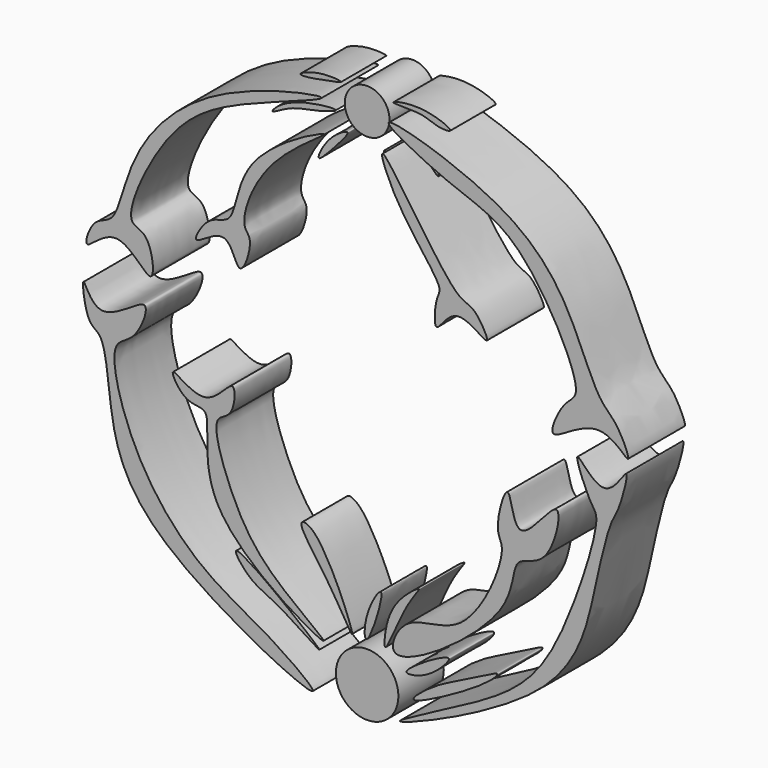
from build123d import *

# Parameters (mm, degrees)
F3_R      = 2.2031193739
F4_DEPTH  = 4
F5_R      = 1.5762828789
F6_DEPTH  = 4
F8_DEPTH  = 5
F13_DEPTH = 5
F14_DEPTH = 5
F15_DEPTH = 5
F19_DEPTH = 5
F20_DEPTH = 5
F21_DEPTH = 5
F22_DEPTH = 5
F29_DEPTH = 4
F30_DEPTH = 4
F31_DEPTH = 4
F32_DEPTH = 4
F33_DEPTH = 4
F34_DEPTH = 4
F39_DEPTH = 4
F40_DEPTH = 4
F41_DEPTH = 4
F42_DEPTH = 4
F45_DEPTH = 4
F46_DEPTH = 4


# Not quite as in the source:
# - the program builds the solid bodies; features that only make, move or delete a surface that nothing else refers to are left out


with BuildPart() as f4:
    # F3 (on Front) → F4 (new body)
    with BuildSketch(Plane.XZ):
        with Locations((0, 2.3418962955)):
            Circle(F3_R)
    extrude(amount=F4_DEPTH)


with BuildPart() as f6:
    # F5 (on Front) → F6 (new body)
    with BuildSketch(Plane.XZ):
        with Locations((0, 37.9213877022)):
            Circle(F5_R)
    extrude(amount=F6_DEPTH)


with BuildPart() as f8:
    # F7 (on Front) → F8 (new body)
    with BuildSketch(Plane.XZ):
        with BuildLine():
            add(Edge.make_bspline(
                [(2.8010457754, 5.6113414466), (3.7490480342, 5.0526232335), (11.660464427, 10.3387411352), (10.7959679961, 14.559460332), (13.7441495824, 14.2067494477), (15.0188095178, 20.4242651347), (11.155763458, 14.1209353977), (10.8886984205, 19.9195584963), (9.6547685549, 15.3268691163), (10.8927378391, 14.7424811012), (7.938159407, 7.593573555), (3.4600012996, 8.6814348962), (2.339180326, 5.8835482227), (2.8010457754, 5.6113414466)],
                knots=[0, 0, 0, 0, 0.1497805879, 0.2426028863, 0.3147246339, 0.4039610203, 0.4935151706, 0.5675421593, 0.6465099561, 0.7028059861, 0.826898522, 0.9270270952, 1, 1, 1, 1], degree=3))
        make_face()
    extrude(amount=F8_DEPTH)


with BuildPart() as f13:
    # F10 (on Front) → F13 (new body)
    with BuildSketch(Plane.XZ):
        with BuildLine():
            add(Edge.make_bspline(
                [(-3.0461507849, 1.3452416752), (-3.4818464728, 1.0746526722), (-15.9466824959, 7.0883957863), (-17.3440535719, 14.0645430033), (-17.6964457302, 18.7752133758), (-19.0105397095, 18.8901683902), (-19.4788265599, 22.8417380605), (-18.2227719071, 18.7192140814), (-13.9632338729, 22.9603577053), (-15.5052584544, 18.8233068375), (-17.6905007654, 18.6818873374), (-15.8132900001, 11.5879474918), (-10.9962366401, 6.1504658227), (-6.6372556078, 4.254425972), (-2.8057086264, 1.4945683859), (-3.0461507849, 1.3452416752)],
                knots=[0, 0, 0, 0, 0.1339251424, 0.241594644, 0.3161355758, 0.3560233968, 0.412737319, 0.4636841603, 0.5330688457, 0.5898577481, 0.638861131, 0.7327648109, 0.8364260377, 0.9260923364, 1, 1, 1, 1], degree=3))
        make_face()
    extrude(amount=F13_DEPTH)


with BuildPart() as f14:
    # F11 (on Front) → F14 (new body)
    with BuildSketch(Plane.XZ):
        with BuildLine():
            add(Edge.make_bspline(
                [(-2.2868220694, 4.7186701559), (-2.6059892866, 4.6507073984), (-12.0999546825, 9.7755638468), (-9.7225185843, 16.8469305379), (-12.0622915375, 16.1343630453), (-13.6245494081, 18.964401828), (-10.4806569975, 15.9435882622), (-8.3487910491, 19.617965915), (-8.5830237681, 16.343588236), (-10.4412698192, 16.3521021675), (-8.5839180053, 10.8751642204), (-6.1482469705, 7.5075225049), (-2.0830393164, 4.7620632021), (-2.2868220694, 4.7186701559)],
                knots=[0, 0, 0, 0, 0.1554468363, 0.2749627788, 0.3349269565, 0.3990039473, 0.4767777833, 0.5543183117, 0.6195590867, 0.6743415246, 0.7823936617, 0.9007498811, 1, 1, 1, 1], degree=3))
        make_face()
    extrude(amount=F14_DEPTH)


with BuildPart() as f15:
    # F12 (on Front) → F15 (new body)
    with BuildSketch(Plane.XZ):
        with BuildLine():
            add(Edge.make_bspline(
                [(3.1202319078, 1.4828173444), (3.4277099811, 1.3932976165), (15.1813481771, 6.1176914834), (16.6875533637, 13.5859063631), (17.8983054266, 18.7917910272), (18.5481634415, 19.4361719166), (19.5950481907, 23.4514253732), (17.598851761, 19.2728908312), (14.8574838152, 23.4901190525), (16.5072711493, 19.2369526839), (17.3805448102, 18.7408839057), (15.1014088235, 11.5459960258), (12.3522853152, 6.5322070241), (7.4192099097, 3.8040285678), (2.9342883779, 1.5369532833), (3.1202319078, 1.4828173444)],
                knots=[0, 0, 0, 0, 0.1271530156, 0.2380593294, 0.3201159226, 0.3626020469, 0.4205450423, 0.4754452226, 0.533326587, 0.5942311074, 0.6345672285, 0.7337673076, 0.8273503335, 0.9231057997, 1, 1, 1, 1], degree=3))
        make_face()
    extrude(amount=F15_DEPTH)


with BuildPart() as f19:
    # F18 (on Front) → F19 (new body)
    with BuildSketch(Plane.XZ):
        with BuildLine():
            add(Edge.make_bspline(
                [(2.322970191, 38.3718237281), (2.5270910425, 38.7261250095), (11.9414135575, 36.0254427021), (15.4403073522, 30.293092001), (17.0726428574, 25.8587327004), (18.4737587842, 25.0532840335), (19.7867006527, 21.928521176), (17.1824421043, 25.4080690427), (12.990501005, 21.4406454045), (14.6318823595, 25.2767119865), (16.4303038149, 25.7301784196), (11.7448821367, 34.6297607631), (7.2388170198, 35.5260575644), (2.1717541082, 38.1093515136), (2.322970191, 38.3718237281)],
                knots=[0, 0, 0, 0, 0.1221092671, 0.2379537302, 0.323282405, 0.3794516036, 0.4358004654, 0.4993232222, 0.5769736094, 0.6387431351, 0.688165312, 0.8080616155, 0.9095394473, 1, 1, 1, 1], degree=3))
        make_face()
    extrude(amount=F19_DEPTH)


with BuildPart() as f20:
    # F17 (on Front) → F20 (new body)
    with BuildSketch(Plane.XZ):
        with BuildLine():
            add(Edge.make_bspline(
                [(1.9492642023, 36.2945869565), (2.5109444115, 35.9835217607), (6.9870378528, 28.5395111667), (8.2735961106, 29.1699334606), (10.0407799206, 26.0465320892), (6.971187526, 29.0233585074), (5.4286092857, 25.7134326681), (5.5973243084, 28.6806268497), (6.3325602319, 29.3568256566), (2.8897882043, 33.0379384873), (1.6250355459, 36.4741486516), (1.9492642023, 36.2945869565)],
                knots=[0, 0, 0, 0, 0.2013367397, 0.2860860069, 0.3773616619, 0.480397428, 0.5740353547, 0.6631838563, 0.7269218084, 0.8837788131, 1, 1, 1, 1], degree=3))
        make_face()
    extrude(amount=F20_DEPTH)


with BuildPart() as f21:
    # F16 (on Front) → F21 (new body)
    with BuildSketch(Plane.XZ):
        with BuildLine():
            add(Edge.make_bspline(
                [(-2.4252030998, 38.3797101676), (-2.4789846343, 38.5840722079), (-10.8069291148, 36.8788326973), (-16.0797222373, 30.7867074955), (-16.7930252537, 25.7173030694), (-18.5509802615, 25.8142728569), (-19.4827202682, 22.8675548903), (-16.7471027116, 26.3270879047), (-13.9220735744, 21.7701284075), (-14.4697933803, 26.2085478406), (-16.7366984942, 25.9222789509), (-13.3311489117, 33.4451286462), (-8.560655082, 36.1864951779), (-2.3784401481, 38.2020177249), (-2.4252030998, 38.3797101676)],
                knots=[0, 0, 0, 0, 0.1142575183, 0.2418402879, 0.3288066955, 0.3788868359, 0.4314786293, 0.4961302535, 0.5681089731, 0.6329376534, 0.6802608121, 0.787273635, 0.9006532842, 1, 1, 1, 1], degree=3))
        make_face()
    extrude(amount=F21_DEPTH)


with BuildPart() as f22:
    # F9 (on Front) → F22 (new body)
    with BuildSketch(Plane.XZ):
        with BuildLine():
            add(Edge.make_bspline(
                [(-2.2471314296, 36.1804254353), (-2.4297902392, 36.2355529609), (-8.5531195322, 33.3510451306), (-8.3437817698, 28.2841304607), (-10.4221559056, 28.6321210069), (-11.986198059, 25.7036030989), (-8.902264517, 28.6096428837), (-8.2729905956, 24.6368009538), (-7.1236667489, 28.0723362786), (-8.3168221546, 28.5557775169), (-6.683407476, 33.4905561644), (-2.0860682132, 36.1318155894), (-2.2471314296, 36.1804254353)],
                knots=[0, 0, 0, 0, 0.1469308705, 0.2724688016, 0.3476298065, 0.4252506236, 0.5116434508, 0.5939968645, 0.6788859293, 0.7369512488, 0.8704406393, 1, 1, 1, 1], degree=3))
        make_face()
    extrude(amount=F22_DEPTH)


with BuildPart() as f29:
    # F25 (on Front) → F29 (new body)
    with BuildSketch(Plane.XZ):
        with BuildLine():
            add(Edge.make_bspline(
                [(-1.8493793905, 39.138160646), (-1.8212072767, 39.2195451719), (-3.3926815622, 39.3771778296), (-5.3397557879, 38.5319502967), (-3.4896675647, 38.7516512444), (-2.9207049201, 38.9460915409), (-1.8713033434, 39.0748260119), (-1.8493793905, 39.138160646)],
                knots=[0, 0, 0, 0, 0.229458845, 0.4515464705, 0.6414348687, 0.8214317548, 1, 1, 1, 1], degree=3))
        make_face()
    extrude(amount=F29_DEPTH)


with BuildPart() as f30:
    # F26 (on Front) → F30 (new body)
    with BuildSketch(Plane.XZ):
        with BuildLine():
            add(Edge.make_bspline(
                [(-2.2203600965, 37.2760854661), (-2.2482048938, 37.3740834609), (-4.3006399089, 37.1876575574), (-6.1438132913, 36.4548829278), (-6.9987236159, 35.4434833858), (-5.3279235742, 36.5584028629), (-3.5918143504, 36.7183597714), (-2.1977171419, 37.196395026), (-2.2203600965, 37.2760854661)],
                knots=[0, 0, 0, 0, 0.1813484263, 0.3912494782, 0.4973853163, 0.650377817, 0.8525302895, 1, 1, 1, 1], degree=3))
        make_face()
    extrude(amount=F30_DEPTH)


with BuildPart() as f31:
    # F27 (on Front) → F31 (new body)
    with BuildSketch(Plane.XZ):
        with BuildLine():
            add(Edge.make_bspline(
                [(-1.3842144981, 36.1581631005), (-1.4654348488, 36.2598773586), (-2.8320166984, 35.4910009057), (-3.8049234588, 33.3224757949), (-2.3854156249, 34.8318687171), (-1.2984933507, 36.0508123832), (-1.3842144981, 36.1581631005)],
                knots=[0, 0, 0, 0, 0.247607324, 0.5036170042, 0.7386716047, 1, 1, 1, 1], degree=3))
        make_face()
    extrude(amount=F31_DEPTH)


with BuildPart() as f32:
    # F24 (on Front) → F32 (new body)
    with BuildSketch(Plane.XZ):
        with BuildLine():
            add(Edge.make_bspline(
                [(1.2257457711, 35.8971096575), (1.3447218931, 35.9440675201), (2.3119158995, 34.5374387809), (2.3400667486, 32.9646713994), (1.9558439298, 34.006873836), (1.439716885, 34.8077793744), (1.1374107412, 35.8622453156), (1.2257457711, 35.8971096575)],
                knots=[0, 0, 0, 0, 0.2498050049, 0.4532304733, 0.5993389115, 0.8145297375, 1, 1, 1, 1], degree=3))
        make_face()
    extrude(amount=F32_DEPTH)


with BuildPart() as f33:
    # F28 (on Front) → F33 (new body)
    with BuildSketch(Plane.XZ):
        with BuildLine():
            add(Edge.make_bspline(
                [(1.854308648, 39.066825062), (1.7829226729, 39.1471854731), (3.7626423728, 39.6518215727), (6.5607006963, 38.5445827834), (4.8477423703, 38.5270656292), (3.9337949577, 39.1324017282), (1.9249394007, 38.9873148177), (1.854308648, 39.066825062)],
                knots=[0, 0, 0, 0, 0.2162198195, 0.4547725674, 0.5953127328, 0.7860676614, 1, 1, 1, 1], degree=3))
        make_face()
    extrude(amount=F33_DEPTH)


with BuildPart() as f34:
    # F23 (on Front) → F34 (new body)
    with BuildSketch(Plane.XZ):
        with BuildLine():
            add(Edge.make_bspline(
                [(2.4007428437, 37.5778712332), (2.4898800691, 37.6262023146), (4.923256046, 36.5808170939), (5.1721828368, 35.106890813), (4.2680461742, 36.4346272144), (2.3199123661, 37.5340441523), (2.4007428437, 37.5778712332)],
                knots=[0, 0, 0, 0, 0.3154577662, 0.4986855814, 0.7139399188, 1, 1, 1, 1], degree=3))
        make_face()
    extrude(amount=F34_DEPTH)


with BuildPart() as f39:
    # F38 (on Front) → F39 (new body)
    with BuildSketch(Plane.XZ):
        with BuildLine():
            add(Edge.make_bspline(
                [(-1.0570976883, 5.1477327943), (-1.0093984648, 5.4333380409), (-3.1351298314, 10.7771894873), (-4.936376624, 11.1450995172), (-4.0948741306, 9.6111760638), (-2.5223229035, 7.6437517034), (-1.0877936906, 4.9639365255), (-1.0570976883, 5.1477327943)],
                knots=[0, 0, 0, 0, 0.3072930417, 0.4408190935, 0.5728505652, 0.8022469295, 1, 1, 1, 1], degree=3))
        make_face()
    extrude(amount=F39_DEPTH)


with BuildPart() as f40:
    # F37 (on Front) → F40 (new body)
    with BuildSketch(Plane.XZ):
        with BuildLine():
            add(Edge.make_bspline(
                [(1.2949332595, 5.0863754004), (1.4939007591, 5.1186163463), (2.5944083027, 8.205514), (4.2367450306, 9.9853359657), (1.923911231, 8.2854649724), (1.2535563048, 6.3700668464), (1.1884872267, 5.0691267503), (1.2949332595, 5.0863754004)],
                knots=[0, 0, 0, 0, 0.2651000904, 0.442940017, 0.6326829059, 0.8581735562, 1, 1, 1, 1], degree=3))
        make_face()
    extrude(amount=F40_DEPTH)


with BuildPart() as f41:
    # F35 (on Front) → F41 (new body)
    with BuildSketch(Plane.XZ):
        with BuildLine():
            add(Edge.make_bspline(
                [(3.2992735505, 2.4684630334), (3.6204000545, 2.3474509242), (8.2908014988, 4.8284273099), (9.6323287724, 6.3865119684), (7.2513691654, 4.9850305086), (4.6604319274, 3.9283494495), (3.1320363131, 2.5314840877), (3.2992735505, 2.4684630334)],
                knots=[0, 0, 0, 0, 0.2974666521, 0.4392848746, 0.6076140264, 0.8450844122, 1, 1, 1, 1], degree=3))
        make_face()
    extrude(amount=F41_DEPTH)


with BuildPart() as f42:
    # F36 (on Front) → F42 (new body)
    with BuildSketch(Plane.XZ):
        with BuildLine():
            add(Edge.make_bspline(
                [(-3.368223086, 3.4092757851), (-3.3130259817, 3.4892108713), (-7.4121647777, 6.7965884216), (-9.8398102074, 8.1456007912), (-8.1743390146, 5.9568237641), (-6.5351459029, 5.5384033726), (-3.4120597712, 3.3457925779), (-3.368223086, 3.4092757851)],
                knots=[0, 0, 0, 0, 0.2771037709, 0.4438851386, 0.5939525495, 0.7799284778, 1, 1, 1, 1], degree=3))
        make_face()
    extrude(amount=F42_DEPTH)


with BuildPart() as f45:
    # F44 (on Front) → F45 (new body)
    with BuildSketch(Plane.XZ):
        with BuildLine():
            add(Edge.make_bspline(
                [(2.7825199068, 4.0709096938), (2.9293722277, 4.4577308107), (6.5550985197, 6.6304764507), (5.0606111558, 4.8073786471), (3.741498474, 3.9900895749), (2.7176091072, 3.8999292979), (2.7825199068, 4.0709096938)],
                knots=[0, 0, 0, 0, 0.3657337783, 0.555744446, 0.8383405055, 1, 1, 1, 1], degree=3))
        make_face()
    extrude(amount=F45_DEPTH)


with BuildPart() as f46:
    # F43 (on Front) → F46 (new body)
    with BuildSketch(Plane.XZ):
        with BuildLine():
            add(Edge.make_bspline(
                [(0, 5.1757181063), (0.33455156, 5.448997402), (1.7246378221, 9.9141937408), (-0.2688630303, 6.773433993), (-0.2244292866, 4.9923924707), (0, 5.1757181063)],
                knots=[0, 0, 0, 0, 0.4103762008, 0.7247048018, 1, 1, 1, 1], degree=3))
        make_face()
    extrude(amount=F46_DEPTH)


solid = Compound([f4.part, f6.part, f8.part, f13.part, f14.part, f15.part, f19.part, f20.part, f21.part, f22.part, f29.part, f30.part, f31.part, f32.part, f33.part, f34.part, f39.part, f40.part, f41.part, f42.part, f45.part, f46.part])
